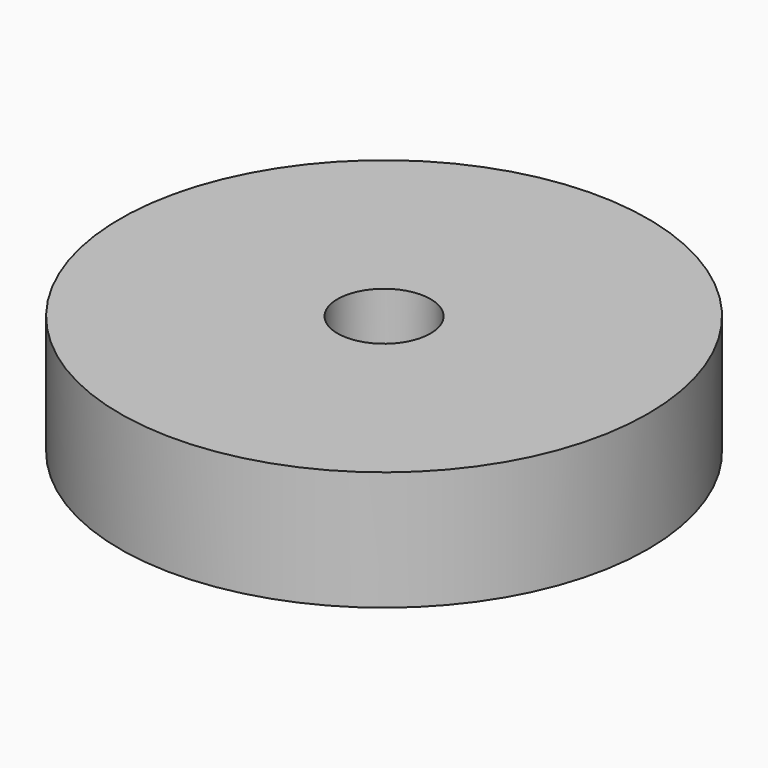
from build123d import *

# Parameters (mm, degrees)
F0_R          = 56.2453252519
F1_DEPTH      = 25.4
F2_R          = 9.9172889071
F3_DEPTH      = 174
F3_DEPTH_BACK = 25.4


# Not quite as in the source:
# - an extrude ends at something that could not be found from the text; its depth is read off the source's solid


with BuildPart() as f1:
    # F0 (on Top) → F1 (new body)
    with BuildSketch(Plane.XY):
        Circle(F0_R)
    extrude(amount=F1_DEPTH)

    # F2 (on Top) → F3 (cut, two sides)
    with BuildSketch(Plane.XY) as f3_sk:
        Circle(F2_R)
    extrude(amount=-F3_DEPTH, mode=Mode.SUBTRACT)
    extrude(f3_sk.sketch, amount=F3_DEPTH_BACK, mode=Mode.SUBTRACT)


solid = f1.part
